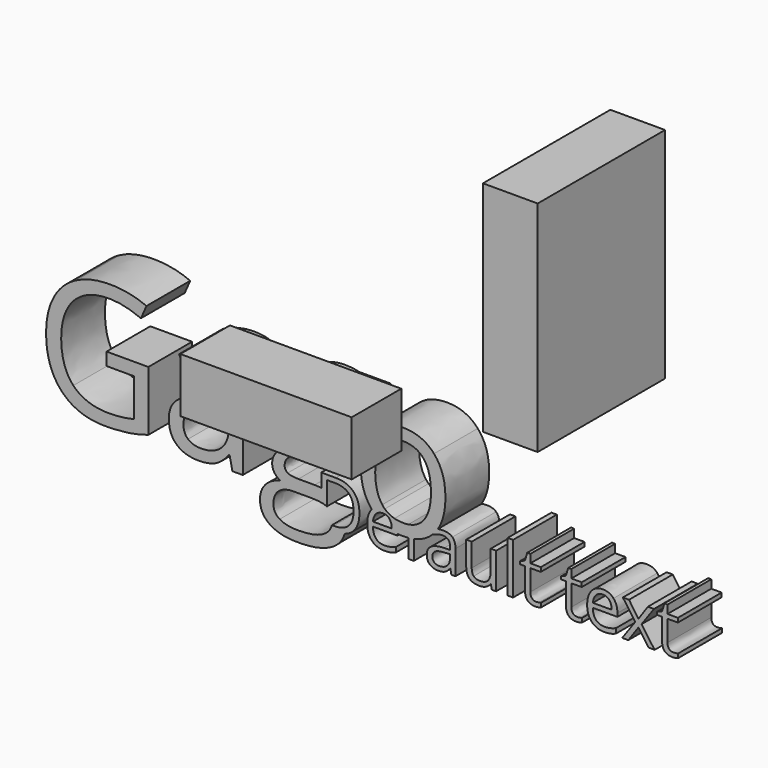
from build123d import *

# Parameters (mm, degrees)
F1_E0_W  = 73.931671679
F1_E0_H  = 101.6
F2_DEPTH = 25.4
F4_W     = 79.559661448
F4_H     = 28.7814624608
F5_DEPTH = 25.4
F6_W     = 2.517619796
F6_H     = 23.5899519612
F7_DEPTH = 25.4


with BuildPart() as f2:
    # F1_E0 (on explicit) → F2 (new body)
    with BuildSketch(Plane(origin=(39.2252579331, 73.931671679, 0), x_dir=(0, -1, 0), z_dir=(-1, 0, 0))):
        with Locations((36.9658358395, 50.8)):
            Rectangle(F1_E0_W, F1_E0_H)
    extrude(amount=F2_DEPTH)


with BuildPart() as f5:
    # F4 (on face) → F5 (new body)
    with BuildSketch(Plane.XY):
        with Locations((-39.779830724, -44.4971304387)):
            Rectangle(F4_W, F4_H)
    extrude(amount=F5_DEPTH)


with BuildPart() as f7:
    # F6 (on Front) → F7 (new body)
    with BuildSketch(Plane.XZ):
        with BuildLine():
            Line((-121.2112891177, -7.0626065135), (-140.6147968438, -7.0626065135))
            Line((-140.6147968438, -7.0626065135), (-140.6147968438, -12.99735614))
            Line((-140.6147968438, -12.99735614), (-127.8582086994, -12.99735614))
            Line((-127.8582086994, -12.99735614), (-127.8582086994, -30.5642150342))
            add(Edge.make_bspline(
                [(-139.452835338, -31.9385781056), (-133.5180857115, -31.9385781056), (-127.8582086994, -30.5642150342)],
                knots=[0, 0, 0, 1, 1, 1], degree=2))
            add(Edge.make_bspline(
                [(-156.026404558, -25.96634585), (-150.3852688604, -31.9385781056), (-139.452835338, -31.9385781056)],
                knots=[0, 0, 0, 1, 1, 1], degree=2))
            add(Edge.make_bspline(
                [(-161.6675402555, -8.4369695849), (-161.6675402555, -19.9941135943), (-156.026404558, -25.96634585)],
                knots=[0, 0, 0, 1, 1, 1], degree=2))
            add(Edge.make_bspline(
                [(-155.8077558875, 8.7862985416), (-161.6675402555, 2.5829234057), (-161.6675402555, -8.4369695849)],
                knots=[0, 0, 0, 1, 1, 1], degree=2))
            add(Edge.make_bspline(
                [(-139.5278005964, 14.9896736774), (-149.9479715195, 14.9896736774), (-155.8077558875, 8.7862985416)],
                knots=[0, 0, 0, 1, 1, 1], degree=2))
            add(Edge.make_bspline(
                [(-124.6471967962, 11.7161907256), (-132.3811126252, 14.9896736774), (-139.5278005964, 14.9896736774)],
                knots=[0, 0, 0, 1, 1, 1], degree=2))
            Line((-124.6471967962, 11.7161907256), (-122.0733895898, 17.5759750936))
            add(Edge.make_bspline(
                [(-139.1029974653, 20.9244233039), (-129.9572359357, 20.9244233039), (-122.0733895898, 17.5759750936)],
                knots=[0, 0, 0, 1, 1, 1], degree=2))
            add(Edge.make_bspline(
                [(-154.8269604229, 17.3948090523), (-148.1113226877, 20.9244233039), (-139.1029974653, 20.9244233039)],
                knots=[0, 0, 0, 1, 1, 1], degree=2))
            add(Edge.make_bspline(
                [(-165.1159421437, 7.1682983802), (-161.5425981581, 13.8651948008), (-154.8269604229, 17.3948090523)],
                knots=[0, 0, 0, 1, 1, 1], degree=2))
            add(Edge.make_bspline(
                [(-168.6892861293, -8.4369695849), (-168.6892861293, 0.4714019597), (-165.1159421437, 7.1682983802)],
                knots=[0, 0, 0, 1, 1, 1], degree=2))
            add(Edge.make_bspline(
                [(-161.4676328997, -30.04570533), (-168.6892861293, -22.3305308157), (-168.6892861293, -8.4369695849)],
                knots=[0, 0, 0, 1, 1, 1], degree=2))
            add(Edge.make_bspline(
                [(-141.2894841697, -37.7608798444), (-154.24597967, -37.7608798444), (-161.4676328997, -30.04570533)],
                knots=[0, 0, 0, 1, 1, 1], degree=2))
            add(Edge.make_bspline(
                [(-130.4320159058, -37.0174743649), (-135.1173445582, -37.7608798444), (-141.2894841697, -37.7608798444)],
                knots=[0, 0, 0, 1, 1, 1], degree=2))
            add(Edge.make_bspline(
                [(-121.2112891177, -34.8247405556), (-125.7466872533, -36.2740688854), (-130.4320159058, -37.0174743649)],
                knots=[0, 0, 0, 1, 1, 1], degree=2))
            Line((-121.2112891177, -34.8247405556), (-121.2112891177, -7.0626065135))
        make_face()
        with BuildLine():
            Line((-83.4662814935, -30.8765702777), (-82.1793778903, -36.9737446308))
            Line((-82.1793778903, -36.9737446308), (-77.3691071404, -36.9737446308))
            Line((-77.3691071404, -36.9737446308), (-77.3691071404, -7.7622822589))
            add(Edge.make_bspline(
                [(-81.0611461186, 3.1264215294), (-77.3691071404, -0.265756415), (-77.3691071404, -7.7622822589)],
                knots=[0, 0, 0, 1, 1, 1], degree=2))
            add(Edge.make_bspline(
                [(-92.3996414575, 6.5185994738), (-84.7531850967, 6.5185994738), (-81.0611461186, 3.1264215294)],
                knots=[0, 0, 0, 1, 1, 1], degree=2))
            add(Edge.make_bspline(
                [(-99.964885455, 5.5440511141), (-96.1978812185, 6.5185994738), (-92.3996414575, 6.5185994738)],
                knots=[0, 0, 0, 1, 1, 1], degree=2))
            add(Edge.make_bspline(
                [(-106.8929247558, 2.85779602), (-103.7318896916, 4.5695027543), (-99.964885455, 5.5440511141)],
                knots=[0, 0, 0, 1, 1, 1], degree=2))
            Line((-106.8929247558, 2.85779602), (-104.8938511974, -2.1024052468))
            add(Edge.make_bspline(
                [(-92.7994561692, 1.1710777051), (-98.1469779379, 1.1710777051), (-104.8938511974, -2.1024052468)],
                knots=[0, 0, 0, 1, 1, 1], degree=2))
            add(Edge.make_bspline(
                [(-85.8651697636, -1.227810565), (-88.0266680486, 1.1710777051), (-92.7994561692, 1.1710777051)],
                knots=[0, 0, 0, 1, 1, 1], degree=2))
            add(Edge.make_bspline(
                [(-83.7036714786, -8.6618653602), (-83.7036714786, -3.626698835), (-85.8651697636, -1.227810565)],
                knots=[0, 0, 0, 1, 1, 1], degree=2))
            Line((-83.7036714786, -8.6618653602), (-83.7036714786, -11.3231320348))
            Line((-83.7036714786, -11.3231320348), (-90.9628073374, -11.5605220199))
            add(Edge.make_bspline(
                [(-111.6907012959, -25.1417280071), (-111.6907012959, -12.1852325069), (-90.9628073374, -11.5605220199)],
                knots=[0, 0, 0, 1, 1, 1], degree=2))
            add(Edge.make_bspline(
                [(-108.0798746811, -34.4749026828), (-111.6907012959, -31.1889255212), (-111.6907012959, -25.1417280071)],
                knots=[0, 0, 0, 1, 1, 1], degree=2))
            add(Edge.make_bspline(
                [(-98.1094953087, -37.7608798444), (-104.4690480663, -37.7608798444), (-108.0798746811, -34.4749026828)],
                knots=[0, 0, 0, 1, 1, 1], degree=2))
            add(Edge.make_bspline(
                [(-90.1569308092, -36.3302928292), (-93.336707188, -37.7608798444), (-98.1094953087, -37.7608798444)],
                knots=[0, 0, 0, 1, 1, 1], degree=2))
            add(Edge.make_bspline(
                [(-83.778636737, -30.8765702777), (-86.9771544304, -34.899705814), (-90.1569308092, -36.3302928292)],
                knots=[0, 0, 0, 1, 1, 1], degree=2))
            Line((-83.778636737, -30.8765702777), (-83.4662814935, -30.8765702777))
        make_face()
        with BuildLine():
            add(Edge.make_bspline(
                [(-96.8225917055, -32.400863866), (-90.7628999816, -32.400863866), (-87.3082509885, -29.0836511801)],
                knots=[0, 0, 0, 1, 1, 1], degree=2))
            add(Edge.make_bspline(
                [(-102.7698355416, -30.5704621391), (-100.6458198859, -32.400863866), (-96.8225917055, -32.400863866)],
                knots=[0, 0, 0, 1, 1, 1], degree=2))
            add(Edge.make_bspline(
                [(-104.8938511974, -25.2166932656), (-104.8938511974, -28.7400604122), (-102.7698355416, -30.5704621391)],
                knots=[0, 0, 0, 1, 1, 1], degree=2))
            add(Edge.make_bspline(
                [(-101.4829319384, -18.6010092083), (-104.8938511974, -20.7312719689), (-104.8938511974, -25.2166932656)],
                knots=[0, 0, 0, 1, 1, 1], degree=2))
            add(Edge.make_bspline(
                [(-90.3380968504, -16.1958738334), (-98.0720126794, -16.4707464476), (-101.4829319384, -18.6010092083)],
                knots=[0, 0, 0, 1, 1, 1], degree=2))
            Line((-90.3380968504, -16.1958738334), (-83.8536019954, -15.9334954288))
            Line((-83.8536019954, -15.9334954288), (-83.8536019954, -19.7942062385))
            add(Edge.make_bspline(
                [(-87.3082509885, -29.0836511801), (-83.8536019954, -25.7664384941), (-83.8536019954, -19.7942062385)],
                knots=[0, 0, 0, 1, 1, 1], degree=2))
        make_face(mode=Mode.SUBTRACT)
        with BuildLine():
            Line((-29.0040212373, 1.7208229336), (-29.0040212373, 5.8189237283))
            Line((-29.0040212373, 5.8189237283), (-43.7971655693, 5.8189237283))
            add(Edge.make_bspline(
                [(-49.8568572932, 6.6060589419), (-46.4959148731, 6.6060589419), (-43.7971655693, 5.8189237283)],
                knots=[0, 0, 0, 1, 1, 1], degree=2))
            add(Edge.make_bspline(
                [(-61.7950746997, 2.7953249713), (-57.5782789124, 6.6060589419), (-49.8568572932, 6.6060589419)],
                knots=[0, 0, 0, 1, 1, 1], degree=2))
            add(Edge.make_bspline(
                [(-66.0118704869, -8.0371548732), (-66.0118704869, -1.0154089994), (-61.7950746997, 2.7953249713)],
                knots=[0, 0, 0, 1, 1, 1], degree=2))
            add(Edge.make_bspline(
                [(-63.9253374603, -15.539927822), (-66.0118704869, -12.2601977653), (-66.0118704869, -8.0371548732)],
                knots=[0, 0, 0, 1, 1, 1], degree=2))
            add(Edge.make_bspline(
                [(-58.5153446429, -20.1815267404), (-61.8388044337, -18.8196578787), (-63.9253374603, -15.539927822)],
                knots=[0, 0, 0, 1, 1, 1], degree=2))
            add(Edge.make_bspline(
                [(-62.4635149207, -23.5799517896), (-61.2140939467, -21.8182682163), (-58.5153446429, -20.1815267404)],
                knots=[0, 0, 0, 1, 1, 1], degree=2))
            add(Edge.make_bspline(
                [(-63.7129358947, -27.6780525843), (-63.7129358947, -25.341635363), (-62.4635149207, -23.5799517896)],
                knots=[0, 0, 0, 1, 1, 1], degree=2))
            add(Edge.make_bspline(
                [(-62.6009512279, -31.3138676186), (-63.7129358947, -29.7520914012), (-63.7129358947, -27.6780525843)],
                knots=[0, 0, 0, 1, 1, 1], degree=2))
            add(Edge.make_bspline(
                [(-59.8522250851, -33.6128022108), (-61.488966561, -32.8756438361), (-62.6009512279, -31.3138676186)],
                knots=[0, 0, 0, 1, 1, 1], degree=2))
            add(Edge.make_bspline(
                [(-66.8739709589, -37.4797601253), (-64.3751290109, -34.6248331997), (-59.8522250851, -33.6128022108)],
                knots=[0, 0, 0, 1, 1, 1], degree=2))
            add(Edge.make_bspline(
                [(-69.3728129069, -44.2328804897), (-69.3728129069, -40.3346870508), (-66.8739709589, -37.4797601253)],
                knots=[0, 0, 0, 1, 1, 1], degree=2))
            add(Edge.make_bspline(
                [(-64.8249205616, -53.0662867758), (-69.3728129069, -49.9427343408), (-69.3728129069, -44.2328804897)],
                knots=[0, 0, 0, 1, 1, 1], degree=2))
            add(Edge.make_bspline(
                [(-51.880919271, -56.1898392108), (-60.2770282163, -56.1898392108), (-64.8249205616, -53.0662867758)],
                knots=[0, 0, 0, 1, 1, 1], degree=2))
            add(Edge.make_bspline(
                [(-35.2511261072, -52.4603176034), (-40.9484857486, -56.1898392108), (-51.880919271, -56.1898392108)],
                knots=[0, 0, 0, 1, 1, 1], degree=2))
            add(Edge.make_bspline(
                [(-30.0711224313, -45.5992812036), (-31.2706132842, -49.8546529594), (-35.2511261072, -52.4603176034)],
                knots=[0.3013407835, 0.3013407835, 0.3013407835, 1, 1, 1], degree=2))
            add(Edge.make_bspline(
                [(-30.0711224313, -45.5992812036), (-32.1260777426, -46.2439060211), (-34.7615723634, -46.2439060211)],
                knots=[0.5287948375, 0.5287948375, 0.5287948375, 1, 1, 1], degree=2))
            Line((-34.7615723634, -46.2439060211), (-36.9914277014, -46.2439060211))
            add(Edge.make_bspline(
                [(-39.7240531941, -48.7870199399), (-37.9620675635, -47.6899874852), (-36.9914277014, -46.2439060211)],
                knots=[0, 0, 0, 0.4491215789, 0.4491215789, 0.4491215789], degree=2))
            add(Edge.make_bspline(
                [(-51.8059540126, -51.229637944), (-43.6472350525, -51.229637944), (-39.7240531941, -48.7870199399)],
                knots=[0, 0, 0, 1, 1, 1], degree=2))
            add(Edge.make_bspline(
                [(-60.1958158529, -49.4304717415), (-57.2659236689, -51.229637944), (-51.8059540126, -51.229637944)],
                knots=[0, 0, 0, 1, 1, 1], degree=2))
            add(Edge.make_bspline(
                [(-63.125708037, -44.1579152313), (-63.125708037, -47.6313055389), (-60.1958158529, -49.4304717415)],
                knots=[0, 0, 0, 1, 1, 1], degree=2))
            add(Edge.make_bspline(
                [(-60.6643487182, -38.1044706123), (-63.125708037, -40.2097449534), (-63.125708037, -44.1579152313)],
                knots=[0, 0, 0, 1, 1, 1], degree=2))
            add(Edge.make_bspline(
                [(-53.7925333612, -35.9991962711), (-58.2029893994, -35.9991962711), (-60.6643487182, -38.1044706123)],
                knots=[0, 0, 0, 1, 1, 1], degree=2))
            Line((-53.7925333612, -35.9991962711), (-46.021134903, -35.9991962711))
            add(Edge.make_bspline(
                [(-40.9028183397, -36.3590525631), (-42.9563452111, -35.9991962711), (-46.021134903, -35.9991962711)],
                knots=[0.4835856801, 0.4835856801, 0.4835856801, 1, 1, 1], degree=2))
            Line((-40.9028183397, -36.3590525631), (-40.9028183397, -30.334794892))
            add(Edge.make_bspline(
                [(-43.959590296, -30.1768945323), (-42.3440056117, -30.1768945323), (-40.9028183397, -30.334794892)],
                knots=[0, 0, 0, 0.2321484242, 0.2321484242, 0.2321484242], degree=2))
            Line((-43.959590296, -30.1768945323), (-51.5310813983, -30.1768945323))
            add(Edge.make_bspline(
                [(-56.4850355602, -29.3397824797), (-55.0419543352, -30.1768945323), (-51.5310813983, -30.1768945323)],
                knots=[0, 0, 0, 1, 1, 1], degree=2))
            add(Edge.make_bspline(
                [(-57.9281167852, -26.7409868538), (-57.9281167852, -28.5026704272), (-56.4850355602, -29.3397824797)],
                knots=[0, 0, 0, 1, 1, 1], degree=2))
            add(Edge.make_bspline(
                [(-53.7925333612, -21.2435345683), (-57.9281167852, -23.4300212728), (-57.9281167852, -26.7409868538)],
                knots=[0, 0, 0, 1, 1, 1], degree=2))
            add(Edge.make_bspline(
                [(-50.2066951659, -21.5558898118), (-52.1183092561, -21.5558898118), (-53.7925333612, -21.2435345683)],
                knots=[0, 0, 0, 1, 1, 1], degree=2))
            add(Edge.make_bspline(
                [(-38.4121611714, -17.8076268898), (-42.710169322, -21.5558898118), (-50.2066951659, -21.5558898118)],
                knots=[0, 0, 0, 1, 1, 1], degree=2))
            add(Edge.make_bspline(
                [(-34.1141530209, -7.7622822589), (-34.1141530209, -14.0593639678), (-38.4121611714, -17.8076268898)],
                knots=[0, 0, 0, 1, 1, 1], degree=2))
            add(Edge.make_bspline(
                [(-34.976253493, -2.7895867825), (-34.1141530209, -5.0010619064), (-34.1141530209, -7.7622822589)],
                knots=[0, 0, 0, 1, 1, 1], degree=2))
            add(Edge.make_bspline(
                [(-36.9253502124, 0.7837572032), (-35.838353965, -0.5781116585), (-34.976253493, -2.7895867825)],
                knots=[0, 0, 0, 1, 1, 1], degree=2))
            Line((-36.9253502124, 0.7837572032), (-29.0040212373, 1.7208229336))
        make_face()
        with BuildLine():
            add(Edge.make_bspline(
                [(-59.6148351, -7.8872243563), (-59.6148351, -12.372645653), (-57.0785105228, -14.67782735)],
                knots=[0, 0, 0, 1, 1, 1], degree=2))
            add(Edge.make_bspline(
                [(-57.1534757813, -0.5843587634), (-59.6148351, -3.0394709773), (-59.6148351, -7.8872243563)],
                knots=[0, 0, 0, 1, 1, 1], degree=2))
            add(Edge.make_bspline(
                [(-50.1192356977, 1.8707534505), (-54.6921164625, 1.8707534505), (-57.1534757813, -0.5843587634)],
                knots=[0, 0, 0, 1, 1, 1], degree=2))
            add(Edge.make_bspline(
                [(-40.5236826175, -7.7622822589), (-40.5236826175, 1.8707534505), (-50.1192356977, 1.8707534505)],
                knots=[0, 0, 0, 1, 1, 1], degree=2))
            add(Edge.make_bspline(
                [(-50.0067878101, -16.983009047), (-40.5236826175, -16.983009047), (-40.5236826175, -7.7622822589)],
                knots=[0, 0, 0, 1, 1, 1], degree=2))
            add(Edge.make_bspline(
                [(-57.0785105228, -14.67782735), (-54.5421859456, -16.983009047), (-50.0067878101, -16.983009047)],
                knots=[0, 0, 0, 1, 1, 1], degree=2))
        make_face(mode=Mode.SUBTRACT)
        with BuildLine():
            Line((-40.9028183397, -24.0801201871), (-40.9028183397, -30.334794892))
            add(Edge.make_bspline(
                [(-40.9028183397, -30.334794892), (-39.5365325686, -30.4844888415), (-38.3269876814, -30.7760968345)],
                knots=[0.2321484242, 0.2321484242, 0.2321484242, 0.4522316118, 0.4522316118, 0.4522316118], degree=2))
            Line((-38.3269876814, -30.7760968345), (-38.3269876814, -26.3115365766))
            Line((-38.3269876814, -26.3115365766), (-34.5820888712, -26.3115365766))
            add(Edge.make_bspline(
                [(-28.1134067942, -28.5089966298), (-30.289037774, -26.3115365766), (-34.5820888712, -26.3115365766)],
                knots=[0, 0, 0, 1, 1, 1], degree=2))
            add(Edge.make_bspline(
                [(-25.9377758145, -35.0431659269), (-25.9377758145, -30.7064566829), (-28.1134067942, -28.5089966298)],
                knots=[0, 0, 0, 1, 1, 1], degree=2))
            add(Edge.make_bspline(
                [(-28.2589339501, -41.7495423584), (-25.9377758145, -39.4817441799), (-25.9377758145, -35.0431659269)],
                knots=[0, 0, 0, 1, 1, 1], degree=2))
            add(Edge.make_bspline(
                [(-29.5916668249, -42.7587820369), (-28.8509159568, -42.3279155833), (-28.2589339501, -41.7495423584)],
                knots=[0.7449626557, 0.7449626557, 0.7449626557, 1, 1, 1], degree=2))
            add(Edge.make_bspline(
                [(-29.5916668249, -42.7587820369), (-29.6937949516, -44.2606559897), (-30.0711224313, -45.5992812036)],
                knots=[0.0815614324, 0.0815614324, 0.0815614324, 0.3013407835, 0.3013407835, 0.3013407835], degree=2))
            add(Edge.make_bspline(
                [(-26.1900228846, -43.3406392622), (-27.7650149298, -44.8758717362), (-30.0711224313, -45.5992812036)],
                knots=[0, 0, 0, 0.5287948375, 0.5287948375, 0.5287948375], degree=2))
            add(Edge.make_bspline(
                [(-23.2115670951, -34.9509987282), (-23.2115670951, -40.4373725032), (-26.1900228846, -43.3406392622)],
                knots=[0, 0, 0, 1, 1, 1], degree=2))
            add(Edge.make_bspline(
                [(-26.0760266125, -26.9445797045), (-23.2115670951, -29.8090392219), (-23.2115670951, -34.9509987282)],
                knots=[0, 0, 0, 1, 1, 1], degree=2))
            add(Edge.make_bspline(
                [(-34.1115510673, -24.0801201871), (-28.9404861299, -24.0801201871), (-26.0760266125, -26.9445797045)],
                knots=[0, 0, 0, 1, 1, 1], degree=2))
            Line((-34.1115510673, -24.0801201871), (-40.9028183397, -24.0801201871))
        make_face()
        with BuildLine():
            add(Edge.make_bspline(
                [(-40.9028183397, -30.334794892), (-39.5365325686, -30.4844888415), (-38.3269876814, -30.7760968345)],
                knots=[0.2321484242, 0.2321484242, 0.2321484242, 0.4522316118, 0.4522316118, 0.4522316118], degree=2))
            Line((-40.9028183397, -30.334794892), (-40.9028183397, -36.3590525631))
            add(Edge.make_bspline(
                [(-38.3269876814, -37.133096148), (-39.3111298317, -36.6379771453), (-40.9028183397, -36.3590525631)],
                knots=[0.0833129835, 0.0833129835, 0.0833129835, 0.4835856801, 0.4835856801, 0.4835856801], degree=2))
            Line((-38.3269876814, -37.133096148), (-38.3269876814, -30.7760968345))
        make_face()
        with BuildLine():
            add(Edge.make_bspline(
                [(-36.9914277014, -46.2439060211), (-36.3030830869, -45.2183944729), (-36.0127190486, -44.0173405368)],
                knots=[0.4491215789, 0.4491215789, 0.4491215789, 0.767623252, 0.767623252, 0.767623252], degree=2))
            Line((-36.9914277014, -46.2439060211), (-34.7615723634, -46.2439060211))
            add(Edge.make_bspline(
                [(-30.0711224313, -45.5992812036), (-32.1260777426, -46.2439060211), (-34.7615723634, -46.2439060211)],
                knots=[0.5287948375, 0.5287948375, 0.5287948375, 1, 1, 1], degree=2))
            add(Edge.make_bspline(
                [(-29.5916668249, -42.7587820369), (-29.6937949516, -44.2606559897), (-30.0711224313, -45.5992812036)],
                knots=[0.0815614324, 0.0815614324, 0.0815614324, 0.3013407835, 0.3013407835, 0.3013407835], degree=2))
            add(Edge.make_bspline(
                [(-35.1884520205, -44.0173405368), (-31.7553959653, -44.0173405368), (-29.5916668249, -42.7587820369)],
                knots=[0, 0, 0, 0.7449626557, 0.7449626557, 0.7449626557], degree=2))
            Line((-35.1884520205, -44.0173405368), (-36.0127190486, -44.0173405368))
        make_face()
        with BuildLine():
            add(Edge.make_bspline(
                [(16.712292201, -15.5336807172), (16.712292201, -24.1072772503), (13.1810554662, -29.6020374845)],
                knots=[0, 0, 0, 0.8188610828, 0.8188610828, 0.8188610828], degree=2))
            add(Edge.make_bspline(
                [(11.4209943761, 0.6275795814), (16.712292201, -5.3508997791), (16.712292201, -15.5336807172)],
                knots=[0, 0, 0, 1, 1, 1], degree=2))
            add(Edge.make_bspline(
                [(-2.8411460419, 6.6060589419), (6.1296965513, 6.6060589419), (11.4209943761, 0.6275795814)],
                knots=[0, 0, 0, 1, 1, 1], degree=2))
            add(Edge.make_bspline(
                [(-17.3719119694, 0.7650158885), (-12.1368380884, 6.6060589419), (-2.8411460419, 6.6060589419)],
                knots=[0, 0, 0, 1, 1, 1], degree=2))
            add(Edge.make_bspline(
                [(-22.6069858505, -15.5336807172), (-22.6069858505, -5.0760271649), (-17.3719119694, 0.7650158885)],
                knots=[0, 0, 0, 1, 1, 1], degree=2))
            add(Edge.make_bspline(
                [(-20.1831091609, -27.3282147116), (-22.6069858505, -22.2930481864), (-22.6069858505, -15.5336807172)],
                knots=[0, 0, 0, 1, 1, 1], degree=2))
            add(Edge.make_bspline(
                [(-17.4641022106, -31.5375090459), (-19.0462406028, -29.689854036), (-20.1831091609, -27.3282147116)],
                knots=[0.5309709594, 0.5309709594, 0.5309709594, 1, 1, 1], degree=2))
            add(Edge.make_bspline(
                [(-17.4641022106, -31.5375090459), (-15.5065536229, -29.3239487025), (-12.2776267866, -29.3239487025)],
                knots=[0.0325088983, 0.0325088983, 0.0325088983, 1, 1, 1], degree=2))
            add(Edge.make_bspline(
                [(-12.2776267866, -29.3239487025), (-11.8272336064, -29.3239487025), (-11.4039469405, -29.3667830636)],
                knots=[0, 0, 0, 0.1443969586, 0.1443969586, 0.1443969586], degree=2))
            add(Edge.make_bspline(
                [(-12.6053709537, -28.0341375619), (-12.0489773215, -28.762218372), (-11.4039469405, -29.3667830636)],
                knots=[0, 0, 0, 0.1696461668, 0.1696461668, 0.1696461668], degree=2))
            add(Edge.make_bspline(
                [(-15.8851010104, -15.5336807172), (-15.8851010104, -23.7423765163), (-12.6053709537, -28.0341375619)],
                knots=[0, 0, 0, 1, 1, 1], degree=2))
            add(Edge.make_bspline(
                [(-12.6428535829, -3.0832007113), (-15.8851010104, -7.2625138693), (-15.8851010104, -15.5336807172)],
                knots=[0, 0, 0, 1, 1, 1], degree=2))
            add(Edge.make_bspline(
                [(-3.0410533978, 1.0961124467), (-9.4006061554, 1.0961124467), (-12.6428535829, -3.0832007113)],
                knots=[0, 0, 0, 1, 1, 1], degree=2))
            add(Edge.make_bspline(
                [(6.7044301993, -3.1394246552), (3.405958828, 1.0961124467), (-3.0410533978, 1.0961124467)],
                knots=[0, 0, 0, 1, 1, 1], degree=2))
            add(Edge.make_bspline(
                [(10.0029015707, -15.5336807172), (10.0029015707, -7.374961757), (6.7044301993, -3.1394246552)],
                knots=[0, 0, 0, 1, 1, 1], degree=2))
            add(Edge.make_bspline(
                [(6.7044301993, -28.0528788765), (10.0029015707, -23.7798591455), (10.0029015707, -15.5336807172)],
                knots=[0, 0, 0, 1, 1, 1], degree=2))
            add(Edge.make_bspline(
                [(5.217899551, -29.6295557297), (6.0261490941, -28.9315612173), (6.7044301993, -28.0528788765)],
                knots=[0.7943650168, 0.7943650168, 0.7943650168, 1, 1, 1], degree=2))
            Line((5.217899551, -29.6295557297), (6.2625328671, -29.6295557297))
            Line((6.2625328671, -29.6295557297), (6.2625328671, -31.5844705231))
            Line((6.2625328671, -31.5844705231), (2.0325435374, -31.5844705231))
            Line((2.0325435374, -31.5844705231), (2.0325435374, -37.246138067))
            add(Edge.make_bspline(
                [(10.6824933978, -32.6829070167), (7.1660772902, -36.1441409171), (2.0325435374, -37.246138067)],
                knots=[0.0705822201, 0.0705822201, 0.0705822201, 0.7040894161, 0.7040894161, 0.7040894161], degree=2))
            Line((10.6824933978, -32.6829070167), (9.9152644786, -30.7792202608))
            add(Edge.make_bspline(
                [(9.9152644786, -30.7792202608), (11.1425434928, -30.1146462492), (12.605091409, -29.736275644)],
                knots=[0, 0, 0, 1, 1, 1], degree=2))
            add(Edge.make_bspline(
                [(12.605091409, -29.736275644), (12.8928387256, -29.6618335521), (13.1810554662, -29.6020374845)],
                knots=[0, 0, 0, 0.1967438561, 0.1967438561, 0.1967438561], degree=2))
        make_face()
        with BuildLine():
            add(Edge.make_bspline(
                [(13.1810554662, -29.6020374845), (14.3577726063, -29.3579050388), (15.5423145043, -29.3579050388)],
                knots=[0.1967438561, 0.1967438561, 0.1967438561, 1, 1, 1], degree=2))
            add(Edge.make_bspline(
                [(13.1810554662, -29.6020374845), (12.3999163791, -30.8175243847), (11.4459827956, -31.8823541618)],
                knots=[0.8188610828, 0.8188610828, 0.8188610828, 1, 1, 1], degree=2))
            add(Edge.make_bspline(
                [(11.4459827956, -31.8823541618), (11.0742749862, -32.2972735552), (10.6824933978, -32.6829070167)],
                knots=[0, 0, 0, 0.0705822201, 0.0705822201, 0.0705822201], degree=2))
            Line((10.6824933978, -32.6829070167), (10.6914093097, -32.7050296231))
            add(Edge.make_bspline(
                [(15.387085538, -31.4340924621), (13.3108981148, -31.4340924621), (10.6914093097, -32.7050296231)],
                knots=[0, 0, 0, 1, 1, 1], degree=2))
            add(Edge.make_bspline(
                [(18.079337921, -32.3654662595), (17.2401313224, -31.4340924621), (15.387085538, -31.4340924621)],
                knots=[0, 0, 0, 1, 1, 1], degree=2))
            add(Edge.make_bspline(
                [(18.9185445197, -35.2517548502), (18.9185445197, -33.2968400568), (18.079337921, -32.3654662595)],
                knots=[0, 0, 0, 1, 1, 1], degree=2))
            Line((18.9185445197, -35.2517548502), (18.9185445197, -36.2849976567))
            Line((18.9185445197, -36.2849976567), (16.1001686016, -36.3771648554))
            add(Edge.make_bspline(
                [(8.0525168839, -41.6500988019), (8.0525168839, -36.6197101151), (16.1001686016, -36.3771648554)],
                knots=[0, 0, 0, 1, 1, 1], degree=2))
            add(Edge.make_bspline(
                [(9.4544284851, -45.2737249822), (8.0525168839, -43.997936916), (8.0525168839, -41.6500988019)],
                knots=[0, 0, 0, 1, 1, 1], degree=2))
            add(Edge.make_bspline(
                [(13.3254508304, -46.5495130484), (10.8563400863, -46.5495130484), (9.4544284851, -45.2737249822)],
                knots=[0, 0, 0, 1, 1, 1], degree=2))
            add(Edge.make_bspline(
                [(16.4130519867, -45.9940844036), (15.1784966147, -46.5495130484), (13.3254508304, -46.5495130484)],
                knots=[0, 0, 0, 1, 1, 1], degree=2))
            add(Edge.make_bspline(
                [(18.8894390885, -43.8766642862), (17.6476073587, -45.4386557588), (16.4130519867, -45.9940844036)],
                knots=[0, 0, 0, 1, 1, 1], degree=2))
            Line((18.8894390885, -43.8766642862), (19.0107117184, -43.8766642862))
            Line((19.0107117184, -43.8766642862), (19.5103549534, -46.2439060211))
            Line((19.5103549534, -46.2439060211), (21.3779534533, -46.2439060211))
            Line((21.3779534533, -46.2439060211), (21.3779534533, -34.9024896762))
            add(Edge.make_bspline(
                [(19.9445109683, -30.6749257992), (21.3779534533, -31.9919465595), (21.3779534533, -34.9024896762)],
                knots=[0, 0, 0, 1, 1, 1], degree=2))
            add(Edge.make_bspline(
                [(15.5423145043, -29.3579050388), (18.5110684833, -29.3579050388), (19.9445109683, -30.6749257992)],
                knots=[0, 0, 0, 1, 1, 1], degree=2))
        make_face()
        with BuildLine():
            add(Edge.make_bspline(
                [(13.8250940654, -44.4684747199), (16.1777830848, -44.4684747199), (17.5190583711, -43.1805593907)],
                knots=[0, 0, 0, 1, 1, 1], degree=2))
            add(Edge.make_bspline(
                [(11.5160631928, -43.7578171089), (12.3407170759, -44.4684747199), (13.8250940654, -44.4684747199)],
                knots=[0, 0, 0, 1, 1, 1], degree=2))
            add(Edge.make_bspline(
                [(10.6914093097, -41.679204233), (10.6914093097, -43.0471594979), (11.5160631928, -43.7578171089)],
                knots=[0, 0, 0, 1, 1, 1], degree=2))
            add(Edge.make_bspline(
                [(12.0157064278, -39.1106499325), (10.6914093097, -39.9377292682), (10.6914093097, -41.679204233)],
                knots=[0, 0, 0, 1, 1, 1], degree=2))
            add(Edge.make_bspline(
                [(16.3427138614, -38.1768506826), (13.3400035459, -38.2835705968), (12.0157064278, -39.1106499325)],
                knots=[0, 0, 0, 1, 1, 1], degree=2))
            Line((16.3427138614, -38.1768506826), (18.8603336574, -38.0749816735))
            Line((18.8603336574, -38.0749816735), (18.8603336574, -39.5739113786))
            add(Edge.make_bspline(
                [(17.5190583711, -43.1805593907), (18.8603336574, -41.8926440616), (18.8603336574, -39.5739113786)],
                knots=[0, 0, 0, 1, 1, 1], degree=2))
        make_face(mode=Mode.SUBTRACT)
        with BuildLine():
            add(Edge.make_bspline(
                [(13.1810554662, -29.6020374845), (12.3999163791, -30.8175243847), (11.4459827956, -31.8823541618)],
                knots=[0.8188610828, 0.8188610828, 0.8188610828, 1, 1, 1], degree=2))
            add(Edge.make_bspline(
                [(12.605091409, -29.736275644), (12.8928387256, -29.6618335521), (13.1810554662, -29.6020374845)],
                knots=[0, 0, 0, 0.1967438561, 0.1967438561, 0.1967438561], degree=2))
            add(Edge.make_bspline(
                [(9.9152644786, -30.7792202608), (11.1425434928, -30.1146462492), (12.605091409, -29.736275644)],
                knots=[0, 0, 0, 1, 1, 1], degree=2))
            Line((9.9152644786, -30.7792202608), (10.6824933978, -32.6829070167))
            add(Edge.make_bspline(
                [(11.4459827956, -31.8823541618), (11.0742749862, -32.2972735552), (10.6824933978, -32.6829070167)],
                knots=[0, 0, 0, 0.0705822201, 0.0705822201, 0.0705822201], degree=2))
        make_face()
        with BuildLine():
            Line((2.0325435374, -46.2439060211), (2.0325435374, -37.246138067))
            add(Edge.make_bspline(
                [(2.0325435374, -37.246138067), (0.8189238149, -37.5066614296), (-0.4850762586, -37.635327567)],
                knots=[0.7040894161, 0.7040894161, 0.7040894161, 0.8538569767, 0.8538569767, 0.8538569767], degree=2))
            Line((-0.4850762586, -37.635327567), (-0.4850762586, -46.2439060211))
            Line((-0.4850762586, -46.2439060211), (2.0325435374, -46.2439060211))
        make_face()
        with BuildLine():
            add(Edge.make_bspline(
                [(2.0325435374, -37.246138067), (0.8189238149, -37.5066614296), (-0.4850762586, -37.635327567)],
                knots=[0.7040894161, 0.7040894161, 0.7040894161, 0.8538569767, 0.8538569767, 0.8538569767], degree=2))
            Line((2.0325435374, -37.246138067), (2.0325435374, -31.5844705231))
            Line((2.0325435374, -31.5844705231), (6.2625328671, -31.5844705231))
            Line((6.2625328671, -31.5844705231), (6.2625328671, -29.6295557297))
            Line((6.2625328671, -29.6295557297), (5.217899551, -29.6295557297))
            add(Edge.make_bspline(
                [(-0.4850762586, -32.1466848395), (2.900588978, -31.630757063), (5.217899551, -29.6295557297)],
                knots=[0.2047944752, 0.2047944752, 0.2047944752, 0.7943650168, 0.7943650168, 0.7943650168], degree=2))
            Line((-0.4850762586, -32.1466848395), (-0.4850762586, -37.635327567))
        make_face()
        with BuildLine():
            add(Edge.make_bspline(
                [(-0.4850762586, -37.635327567), (-1.7575181168, -37.7608798444), (-3.1160186562, -37.7608798444)],
                knots=[0.8538569767, 0.8538569767, 0.8538569767, 1, 1, 1], degree=2))
            Line((-0.4850762586, -37.635327567), (-0.4850762586, -32.1466848395))
            add(Edge.make_bspline(
                [(-2.9660881393, -32.3258986076), (-1.6611281245, -32.3258986076), (-0.4850762586, -32.1466848395)],
                knots=[0, 0, 0, 0.2047944752, 0.2047944752, 0.2047944752], degree=2))
            add(Edge.make_bspline(
                [(-6.9833499712, -31.8162599346), (-5.1575806752, -32.3258986076), (-2.9660881393, -32.3258986076)],
                knots=[0.6554014694, 0.6554014694, 0.6554014694, 1, 1, 1], degree=2))
            add(Edge.make_bspline(
                [(-6.9833499712, -31.8162599346), (-5.5203158505, -33.7800591314), (-5.5203158505, -36.7991936073)],
                knots=[0.1031905001, 0.1031905001, 0.1031905001, 1, 1, 1], degree=2))
            Line((-5.5203158505, -36.7991936073), (-5.5203158505, -37.6368710395))
            add(Edge.make_bspline(
                [(-3.1160186562, -37.7608798444), (-4.3480212249, -37.7608798444), (-5.5203158505, -37.6368710395)],
                knots=[0, 0, 0, 0.2143606126, 0.2143606126, 0.2143606126], degree=2))
        make_face()
        with BuildLine():
            add(Edge.make_bspline(
                [(-17.4641022106, -31.5375090459), (-15.5065536229, -29.3239487025), (-12.2776267866, -29.3239487025)],
                knots=[0.0325088983, 0.0325088983, 0.0325088983, 1, 1, 1], degree=2))
            add(Edge.make_bspline(
                [(-15.8575239542, -33.1795689188), (-16.7112269885, -32.4167328122), (-17.4641022106, -31.5375090459)],
                knots=[0.307779142, 0.307779142, 0.307779142, 0.5309709594, 0.5309709594, 0.5309709594], degree=2))
            add(Edge.make_bspline(
                [(-15.5010532884, -32.7365605068), (-15.6918308216, -32.9452112917), (-15.8575239542, -33.1795689188)],
                knots=[0, 0, 0, 0.1601964713, 0.1601964713, 0.1601964713], degree=2))
            add(Edge.make_bspline(
                [(-12.3115831229, -31.4340924621), (-14.3101560631, -31.4340924621), (-15.5010532884, -32.7365605068)],
                knots=[0, 0, 0, 1, 1, 1], degree=2))
            add(Edge.make_bspline(
                [(-9.2773419237, -32.7001787179), (-10.3372647087, -31.4340924621), (-12.3115831229, -31.4340924621)],
                knots=[0, 0, 0, 1, 1, 1], degree=2))
            add(Edge.make_bspline(
                [(-8.2174191387, -36.343208519), (-8.2174191387, -33.9662649737), (-9.2773419237, -32.7001787179)],
                knots=[0, 0, 0, 1, 1, 1], degree=2))
            Line((-8.2174191387, -36.343208519), (-10.7645510908, -36.343208519))
            add(Edge.make_bspline(
                [(-5.5203158505, -37.6368710395), (-8.3116985334, -37.3415902943), (-10.7645510908, -36.343208519)],
                knots=[0.2143606126, 0.2143606126, 0.2143606126, 0.7247805095, 0.7247805095, 0.7247805095], degree=2))
            Line((-5.5203158505, -37.6368710395), (-5.5203158505, -36.7991936073))
            add(Edge.make_bspline(
                [(-6.9833499712, -31.8162599346), (-5.5203158505, -33.7800591314), (-5.5203158505, -36.7991936073)],
                knots=[0.1031905001, 0.1031905001, 0.1031905001, 1, 1, 1], degree=2))
            add(Edge.make_bspline(
                [(-11.4039469405, -29.3667830636), (-9.5570031878, -31.0978596347), (-6.9833499712, -31.8162599346)],
                knots=[0.1696461668, 0.1696461668, 0.1696461668, 0.6554014694, 0.6554014694, 0.6554014694], degree=2))
            add(Edge.make_bspline(
                [(-12.2776267866, -29.3239487025), (-11.8272336064, -29.3239487025), (-11.4039469405, -29.3667830636)],
                knots=[0, 0, 0, 0.1443969586, 0.1443969586, 0.1443969586], degree=2))
        make_face()
        with BuildLine():
            add(Edge.make_bspline(
                [(-15.8575239542, -33.1795689188), (-16.7112269885, -32.4167328122), (-17.4641022106, -31.5375090459)],
                knots=[0.307779142, 0.307779142, 0.307779142, 0.5309709594, 0.5309709594, 0.5309709594], degree=2))
            add(Edge.make_bspline(
                [(-17.5942188798, -31.6887649848), (-17.5298782657, -31.6118874128), (-17.4641022106, -31.5375090459)],
                knots=[0, 0, 0, 0.0325088983, 0.0325088983, 0.0325088983], degree=2))
            add(Edge.make_bspline(
                [(-19.5733881992, -38.0749816735), (-19.5733881992, -34.0535812672), (-17.5942188798, -31.6887649848)],
                knots=[0, 0, 0, 1, 1, 1], degree=2))
            add(Edge.make_bspline(
                [(-17.4414153662, -44.3035439433), (-19.5733881992, -42.0575748382), (-19.5733881992, -38.0749816735)],
                knots=[0, 0, 0, 1, 1, 1], degree=2))
            add(Edge.make_bspline(
                [(-11.6276054905, -46.5495130484), (-15.3094425332, -46.5495130484), (-17.4414153662, -44.3035439433)],
                knots=[0, 0, 0, 1, 1, 1], degree=2))
            add(Edge.make_bspline(
                [(-8.7558696153, -46.2972659783), (-9.944341388, -46.5495130484), (-11.6276054905, -46.5495130484)],
                knots=[0, 0, 0, 1, 1, 1], degree=2))
            add(Edge.make_bspline(
                [(-6.2333989141, -45.4726120952), (-7.5673978426, -46.0450189081), (-8.7558696153, -46.2972659783)],
                knots=[0, 0, 0, 1, 1, 1], degree=2))
            Line((-6.2333989141, -45.4726120952), (-6.2333989141, -43.2266429901))
            add(Edge.make_bspline(
                [(-11.5354382918, -44.34720209), (-8.8528877192, -44.34720209), (-6.2333989141, -43.2266429901)],
                knots=[0, 0, 0, 1, 1, 1], degree=2))
            add(Edge.make_bspline(
                [(-15.4840751202, -42.8312942167), (-14.082163519, -44.34720209), (-11.5354382918, -44.34720209)],
                knots=[0, 0, 0, 1, 1, 1], degree=2))
            add(Edge.make_bspline(
                [(-16.9636012045, -38.3902905111), (-16.8859867214, -41.3153863434), (-15.4840751202, -42.8312942167)],
                knots=[0, 0, 0, 1, 1, 1], degree=2))
            Line((-16.9636012045, -38.3902905111), (-5.5203158505, -38.3902905111))
            Line((-5.5203158505, -38.3902905111), (-5.5203158505, -37.6368710395))
            add(Edge.make_bspline(
                [(-5.5203158505, -37.6368710395), (-8.3116985334, -37.3415902943), (-10.7645510908, -36.343208519)],
                knots=[0.2143606126, 0.2143606126, 0.2143606126, 0.7247805095, 0.7247805095, 0.7247805095], degree=2))
            Line((-10.7645510908, -36.343208519), (-16.9053903422, -36.343208519))
            add(Edge.make_bspline(
                [(-15.8575239542, -33.1795689188), (-16.726142821, -34.4081500517), (-16.9053903422, -36.343208519)],
                knots=[0.1601964713, 0.1601964713, 0.1601964713, 1, 1, 1], degree=2))
        make_face()
        with BuildLine():
            Line((28.9259619361, -40.4082670721), (28.9259619361, -29.6295557297))
            Line((28.9259619361, -29.6295557297), (26.3792367089, -29.6295557297))
            Line((26.3792367089, -29.6295557297), (26.3792367089, -40.5004342707))
            add(Edge.make_bspline(
                [(27.8854427719, -45.1087942056), (26.3792367089, -43.6680753628), (26.3792367089, -40.5004342707)],
                knots=[0, 0, 0, 1, 1, 1], degree=2))
            add(Edge.make_bspline(
                [(32.4234645814, -46.5495130484), (29.3916488348, -46.5495130484), (27.8854427719, -45.1087942056)],
                knots=[0, 0, 0, 1, 1, 1], degree=2))
            add(Edge.make_bspline(
                [(35.5571493371, -45.8970662997), (34.184343167, -46.5495130484), (32.4234645814, -46.5495130484)],
                knots=[0, 0, 0, 1, 1, 1], degree=2))
            add(Edge.make_bspline(
                [(37.7012494331, -44.0173405368), (36.9299555071, -45.244619551), (35.5571493371, -45.8970662997)],
                knots=[0, 0, 0, 1, 1, 1], degree=2))
            Line((37.7012494331, -44.0173405368), (37.8370747785, -44.0173405368))
            Line((37.8370747785, -44.0173405368), (38.2008926681, -46.2439060211))
            Line((38.2008926681, -46.2439060211), (40.2770800914, -46.2439060211))
            Line((40.2770800914, -46.2439060211), (40.2770800914, -29.6295557297))
            Line((40.2770800914, -29.6295557297), (37.7594602954, -29.6295557297))
            Line((37.7594602954, -29.6295557297), (37.7594602954, -38.3611850799))
            add(Edge.make_bspline(
                [(36.5564358071, -43.0156286141), (37.7594602954, -41.5918879395), (37.7594602954, -38.3611850799)],
                knots=[0, 0, 0, 1, 1, 1], degree=2))
            add(Edge.make_bspline(
                [(32.7436243242, -44.4393692887), (35.3534113189, -44.4393692887), (36.5564358071, -43.0156286141)],
                knots=[0, 0, 0, 1, 1, 1], degree=2))
            add(Edge.make_bspline(
                [(29.8500593757, -43.4400828187), (30.7741568152, -44.4393692887), (32.7436243242, -44.4393692887)],
                knots=[0, 0, 0, 1, 1, 1], degree=2))
            add(Edge.make_bspline(
                [(28.9259619361, -40.4082670721), (28.9259619361, -42.4407963486), (29.8500593757, -43.4400828187)],
                knots=[0, 0, 0, 1, 1, 1], degree=2))
        make_face()
        with Locations((46.8718857034, -34.4489300405)):
            Rectangle(F6_W, F6_H)
        with BuildLine():
            add(Edge.make_bspline(
                [(58.8317924606, -44.4684747199), (59.5012173774, -44.4684747199), (60.1221332424, -44.371456616)],
                knots=[0, 0, 0, 1, 1, 1], degree=2))
            add(Edge.make_bspline(
                [(56.8768776672, -43.6656499102), (57.5899607308, -44.4684747199), (58.8317924606, -44.4684747199)],
                knots=[0, 0, 0, 1, 1, 1], degree=2))
            add(Edge.make_bspline(
                [(56.1637946036, -41.3638953954), (56.1637946036, -42.8628251005), (56.8768776672, -43.6656499102)],
                knots=[0, 0, 0, 1, 1, 1], degree=2))
            Line((56.1637946036, -41.3638953954), (56.1637946036, -31.5844705231))
            Line((56.1637946036, -31.5844705231), (60.985594367, -31.5844705231))
            Line((60.985594367, -31.5844705231), (60.985594367, -29.6295557297))
            Line((60.985594367, -29.6295557297), (56.1637946036, -29.6295557297))
            Line((56.1637946036, -29.6295557297), (56.1637946036, -25.7779370052))
            Line((56.1637946036, -25.7779370052), (54.7085230452, -25.7779370052))
            Line((54.7085230452, -25.7779370052), (53.6510257128, -29.3239487025))
            Line((53.6510257128, -29.3239487025), (51.2692312623, -30.3717442245))
            Line((51.2692312623, -30.3717442245), (51.2692312623, -31.5844705231))
            Line((51.2692312623, -31.5844705231), (53.6510257128, -31.5844705231))
            Line((53.6510257128, -31.5844705231), (53.6510257128, -41.4706153097))
            add(Edge.make_bspline(
                [(58.467974571, -46.5495130484), (53.6510257128, -46.5495130484), (53.6510257128, -41.4706153097)],
                knots=[0, 0, 0, 1, 1, 1], degree=2))
            add(Edge.make_bspline(
                [(59.9038425086, -46.4185386081), (59.1082940567, -46.5495130484), (58.467974571, -46.5495130484)],
                knots=[0, 0, 0, 1, 1, 1], degree=2))
            add(Edge.make_bspline(
                [(61.1068669969, -46.0935279601), (60.6993909605, -46.2875641679), (59.9038425086, -46.4185386081)],
                knots=[0, 0, 0, 1, 1, 1], degree=2))
            Line((61.1068669969, -46.0935279601), (61.1068669969, -44.1677185978))
            add(Edge.make_bspline(
                [(60.1221332424, -44.371456616), (60.7430491073, -44.2744385121), (61.1068669969, -44.1677185978)],
                knots=[0, 0, 0, 1, 1, 1], degree=2))
        make_face()
        with BuildLine():
            add(Edge.make_bspline(
                [(77.8570426337, -44.4684747199), (78.5264675505, -44.4684747199), (79.1473834155, -44.371456616)],
                knots=[0, 0, 0, 1, 1, 1], degree=2))
            add(Edge.make_bspline(
                [(75.9021278403, -43.6656499102), (76.6152109039, -44.4684747199), (77.8570426337, -44.4684747199)],
                knots=[0, 0, 0, 1, 1, 1], degree=2))
            add(Edge.make_bspline(
                [(75.1890447767, -41.3638953954), (75.1890447767, -42.8628251005), (75.9021278403, -43.6656499102)],
                knots=[0, 0, 0, 1, 1, 1], degree=2))
            Line((75.1890447767, -41.3638953954), (75.1890447767, -31.5844705231))
            Line((75.1890447767, -31.5844705231), (80.0108445401, -31.5844705231))
            Line((80.0108445401, -31.5844705231), (80.0108445401, -29.6295557297))
            Line((80.0108445401, -29.6295557297), (75.1890447767, -29.6295557297))
            Line((75.1890447767, -29.6295557297), (75.1890447767, -25.7779370052))
            Line((75.1890447767, -25.7779370052), (73.7337732183, -25.7779370052))
            Line((73.7337732183, -25.7779370052), (72.6762758859, -29.3239487025))
            Line((72.6762758859, -29.3239487025), (70.2944814354, -30.3717442245))
            Line((70.2944814354, -30.3717442245), (70.2944814354, -31.5844705231))
            Line((70.2944814354, -31.5844705231), (72.6762758859, -31.5844705231))
            Line((72.6762758859, -31.5844705231), (72.6762758859, -41.4706153097))
            add(Edge.make_bspline(
                [(77.4932247441, -46.5495130484), (72.6762758859, -46.5495130484), (72.6762758859, -41.4706153097)],
                knots=[0, 0, 0, 1, 1, 1], degree=2))
            add(Edge.make_bspline(
                [(78.9290926817, -46.4185386081), (78.1335442298, -46.5495130484), (77.4932247441, -46.5495130484)],
                knots=[0, 0, 0, 1, 1, 1], degree=2))
            add(Edge.make_bspline(
                [(80.1321171699, -46.0935279601), (79.7246411336, -46.2875641679), (78.9290926817, -46.4185386081)],
                knots=[0, 0, 0, 1, 1, 1], degree=2))
            Line((80.1321171699, -46.0935279601), (80.1321171699, -44.1677185978))
            add(Edge.make_bspline(
                [(79.1473834155, -44.371456616), (79.7682992804, -44.2744385121), (80.1321171699, -44.1677185978)],
                knots=[0, 0, 0, 1, 1, 1], degree=2))
        make_face()
        with BuildLine():
            add(Edge.make_bspline(
                [(90.4693961396, -46.5495130484), (86.7875590969, -46.5495130484), (84.6555862639, -44.3035439433)],
                knots=[0, 0, 0, 1, 1, 1], degree=2))
            add(Edge.make_bspline(
                [(93.3411320148, -46.2972659783), (92.1526602421, -46.5495130484), (90.4693961396, -46.5495130484)],
                knots=[0, 0, 0, 1, 1, 1], degree=2))
            add(Edge.make_bspline(
                [(95.8636027159, -45.4726120952), (94.5296037874, -46.0450189081), (93.3411320148, -46.2972659783)],
                knots=[0, 0, 0, 1, 1, 1], degree=2))
            Line((95.8636027159, -45.4726120952), (95.8636027159, -43.2266429901))
            add(Edge.make_bspline(
                [(90.5615633383, -44.34720209), (93.2441139109, -44.34720209), (95.8636027159, -43.2266429901)],
                knots=[0, 0, 0, 1, 1, 1], degree=2))
            add(Edge.make_bspline(
                [(86.6129265099, -42.8312942167), (88.0148381111, -44.34720209), (90.5615633383, -44.34720209)],
                knots=[0, 0, 0, 1, 1, 1], degree=2))
            add(Edge.make_bspline(
                [(85.1334004255, -38.3902905111), (85.2110149087, -41.3153863434), (86.6129265099, -42.8312942167)],
                knots=[0, 0, 0, 1, 1, 1], degree=2))
            Line((85.1334004255, -38.3902905111), (96.5766857795, -38.3902905111))
            Line((96.5766857795, -38.3902905111), (96.5766857795, -36.7991936073))
            add(Edge.make_bspline(
                [(94.7575963316, -31.3783070524), (96.5766857795, -33.4326654023), (96.5766857795, -36.7991936073)],
                knots=[0, 0, 0, 1, 1, 1], degree=2))
            add(Edge.make_bspline(
                [(89.8193748435, -29.3239487025), (92.9385068836, -29.3239487025), (94.7575963316, -31.3783070524)],
                knots=[0, 0, 0, 1, 1, 1], degree=2))
            add(Edge.make_bspline(
                [(84.5027827503, -31.6887649848), (86.4819520696, -29.3239487025), (89.8193748435, -29.3239487025)],
                knots=[0, 0, 0, 1, 1, 1], degree=2))
            add(Edge.make_bspline(
                [(82.5236134309, -38.0749816735), (82.5236134309, -34.0535812672), (84.5027827503, -31.6887649848)],
                knots=[0, 0, 0, 1, 1, 1], degree=2))
            add(Edge.make_bspline(
                [(84.6555862639, -44.3035439433), (82.5236134309, -42.0575748382), (82.5236134309, -38.0749816735)],
                knots=[0, 0, 0, 1, 1, 1], degree=2))
        make_face()
        with BuildLine():
            add(Edge.make_bspline(
                [(89.7854185071, -31.4340924621), (87.786845567, -31.4340924621), (86.5959483417, -32.7365605068)],
                knots=[0, 0, 0, 1, 1, 1], degree=2))
            add(Edge.make_bspline(
                [(92.8196597063, -32.7001787179), (91.7597369213, -31.4340924621), (89.7854185071, -31.4340924621)],
                knots=[0, 0, 0, 1, 1, 1], degree=2))
            add(Edge.make_bspline(
                [(93.8795824914, -36.343208519), (93.8795824914, -33.9662649737), (92.8196597063, -32.7001787179)],
                knots=[0, 0, 0, 1, 1, 1], degree=2))
            Line((93.8795824914, -36.343208519), (85.1916112879, -36.343208519))
            add(Edge.make_bspline(
                [(86.5959483417, -32.7365605068), (85.4050511164, -34.0390285516), (85.1916112879, -36.343208519)],
                knots=[0, 0, 0, 1, 1, 1], degree=2))
        make_face(mode=Mode.SUBTRACT)
        Polygon((99.0943055755, -29.6295557297), (104.8717336622, -37.740269215), (98.7935494535, -46.2439060211), (101.6410308027, -46.2439060211), (106.3415579362, -39.5108496111), (110.998426923, -46.2439060211), (113.8459082722, -46.2439060211), (107.7677240634, -37.740269215), (113.5451521501, -29.6295557297), (110.7073726113, -29.6295557297), (106.3415579362, -35.993943345), (101.9611905455, -29.6295557297), align=None)
        with BuildLine():
            add(Edge.make_bspline(
                [(122.4999231393, -44.4684747199), (123.1693480562, -44.4684747199), (123.7902639211, -44.371456616)],
                knots=[0, 0, 0, 1, 1, 1], degree=2))
            add(Edge.make_bspline(
                [(120.5450083459, -43.6656499102), (121.2580914095, -44.4684747199), (122.4999231393, -44.4684747199)],
                knots=[0, 0, 0, 1, 1, 1], degree=2))
            add(Edge.make_bspline(
                [(119.8319252823, -41.3638953954), (119.8319252823, -42.8628251005), (120.5450083459, -43.6656499102)],
                knots=[0, 0, 0, 1, 1, 1], degree=2))
            Line((119.8319252823, -41.3638953954), (119.8319252823, -31.5844705231))
            Line((119.8319252823, -31.5844705231), (124.6537250457, -31.5844705231))
            Line((124.6537250457, -31.5844705231), (124.6537250457, -29.6295557297))
            Line((124.6537250457, -29.6295557297), (119.8319252823, -29.6295557297))
            Line((119.8319252823, -29.6295557297), (119.8319252823, -25.7779370052))
            Line((119.8319252823, -25.7779370052), (118.3766537239, -25.7779370052))
            Line((118.3766537239, -25.7779370052), (117.3191563915, -29.3239487025))
            Line((117.3191563915, -29.3239487025), (114.937361941, -30.3717442245))
            Line((114.937361941, -30.3717442245), (114.937361941, -31.5844705231))
            Line((114.937361941, -31.5844705231), (117.3191563915, -31.5844705231))
            Line((117.3191563915, -31.5844705231), (117.3191563915, -41.4706153097))
            add(Edge.make_bspline(
                [(122.1361052497, -46.5495130484), (117.3191563915, -46.5495130484), (117.3191563915, -41.4706153097)],
                knots=[0, 0, 0, 1, 1, 1], degree=2))
            add(Edge.make_bspline(
                [(123.5719731873, -46.4185386081), (122.7764247354, -46.5495130484), (122.1361052497, -46.5495130484)],
                knots=[0, 0, 0, 1, 1, 1], degree=2))
            add(Edge.make_bspline(
                [(124.7749976756, -46.0935279601), (124.3675216392, -46.2875641679), (123.5719731873, -46.4185386081)],
                knots=[0, 0, 0, 1, 1, 1], degree=2))
            Line((124.7749976756, -46.0935279601), (124.7749976756, -44.1677185978))
            add(Edge.make_bspline(
                [(123.7902639211, -44.371456616), (124.411179786, -44.2744385121), (124.7749976756, -44.1677185978)],
                knots=[0, 0, 0, 1, 1, 1], degree=2))
        make_face()
    extrude(amount=F7_DEPTH)


solid = Compound([f2.part, f5.part, f7.part])
